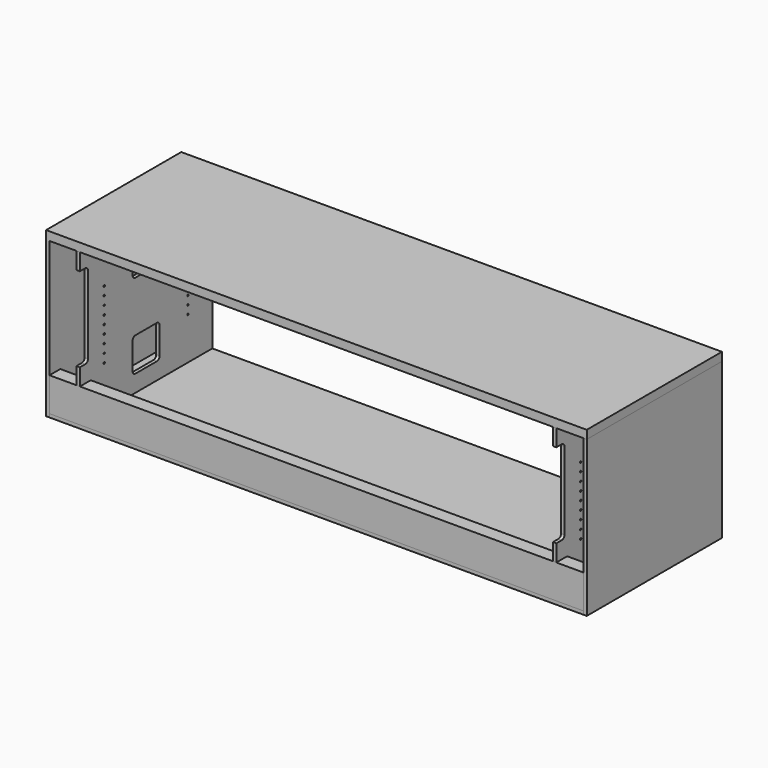
from build123d import *

# Parameters (mm, degrees)
F0_W      = 1600
F0_H      = 500
F1_DEPTH  = 25
F3_W      = 1580
F3_H      = 490
F4_DEPTH  = 10
F5_W      = 10
F5_H      = 500
F6_DEPTH  = 460
F7_W      = 10
F7_H      = 500
F8_DEPTH  = 460
F9_W      = 40
F9_H      = 100
F10_DEPTH = 1580
F11_W     = 10
F11_H     = 450
F12_DEPTH = 450
F13_W     = 10
F13_H     = 350
F14_DEPTH = 40
F16_W     = 30
F16_H     = 250
F17_DEPTH = 100.001
F18_R     = 10
F20_DEPTH = 100.001
F21_R     = 2.5
F22_DEPTH = 100.001


with BuildPart() as f1:
    # F0 (on Top) → F1 (new body)
    with BuildSketch(Plane.XY):
        with Locations((800, 250)):
            Rectangle(F0_W, F0_H)
    extrude(amount=F1_DEPTH)

    # F5 (on face) → F6 (join, through all)
    with BuildSketch(Plane.XY):
        with Locations((5, 250)):
            Rectangle(F5_W, F5_H)
    extrude(amount=-F6_DEPTH)


with BuildPart() as f4:
    # F3 (on offset) → F4 (new body)
    with BuildSketch(Plane.XY.offset(-460)):
        with Locations((800, 245)):
            Rectangle(F3_W, F3_H)
    extrude(amount=F4_DEPTH)


with BuildPart() as f8:
    # F7 (on face) → F8 (new body, through all)
    with BuildSketch(Plane.XY):
        with Locations((1595, 250)):
            Rectangle(F7_W, F7_H)
    extrude(amount=-F8_DEPTH)


with BuildPart() as f10:
    # F9 (on face) → F10 (new body, through all)
    with BuildSketch(Plane.YZ.offset(10)):
        with Locations((20, -400)):
            Rectangle(F9_W, F9_H)
    extrude(amount=F10_DEPTH)


with BuildPart() as f12:
    # F11 (on face) → F12 (new body, through all)
    with BuildSketch(Plane.XY.offset(-450)):
        with Locations((95, 265)):
            Rectangle(F11_W, F11_H)
    extrude(amount=F12_DEPTH)

    # F13 (on face) → F14 (join, through all)
    with BuildSketch(Plane.XZ.offset(-40)):
        with Locations((95, -175)):
            Rectangle(F13_W, F13_H)
    extrude(amount=F14_DEPTH)

    # F15: union 

    # F16 (on face) → F17 (cut, through all)
    with BuildSketch(Plane.YZ.offset(100)):
        with Locations((15, -175)):
            Rectangle(F16_W, F16_H)
    extrude(amount=-F17_DEPTH, mode=Mode.SUBTRACT)

    # F18
    f18_edges = [f12.edges().sort_by_distance(p)[0] for p in [
        (95, 30, -50),
        (95, 30, -300),
    ]]
    fillet(f18_edges, radius=F18_R)

    # F19 (on face) → F20 (cut, through all)
    with BuildSketch(Plane.YZ.offset(100)):
        with BuildLine():
            Line((285, -50), (205, -50))
            ThreePointArc((205, -50), (197.9289321881, -52.9289321881), (195, -60))
            Line((195, -60), (195, -140))
            ThreePointArc((195, -140), (197.9289321881, -147.0710678119), (205, -150))
            Line((205, -150), (285, -150))
            ThreePointArc((285, -150), (292.0710678119, -147.0710678119), (295, -140))
            Line((295, -140), (295, -60))
            ThreePointArc((295, -60), (292.0710678119, -52.9289321881), (285, -50))
        make_face()
        with BuildLine():
            Line((285, -300), (205, -300))
            ThreePointArc((205, -300), (197.9289321881, -302.9289321881), (195, -310))
            Line((195, -310), (195, -390))
            ThreePointArc((195, -390), (197.9289321881, -397.0710678119), (205, -400))
            Line((205, -400), (285, -400))
            ThreePointArc((285, -400), (292.0710678119, -397.0710678119), (295, -390))
            Line((295, -390), (295, -310))
            ThreePointArc((295, -310), (292.0710678119, -302.9289321881), (285, -300))
        make_face()
    extrude(amount=-F20_DEPTH, mode=Mode.SUBTRACT)

    # F21 (on face) → F22 (cut, through all)
    with BuildSketch(Plane.YZ.offset(100)):
        with Locations((90, -325)):
            Circle(F21_R)
        with Locations((90, -300)):
            Circle(F21_R)
        with Locations((90, -275)):
            Circle(F21_R)
        with Locations((90, -250)):
            Circle(F21_R)
        with Locations((90, -225)):
            Circle(F21_R)
        with Locations((90, -200)):
            Circle(F21_R)
        with Locations((90, -175)):
            Circle(F21_R)
        with Locations((90, -150)):
            Circle(F21_R)
        with Locations((90, -125)):
            Circle(F21_R)
        with Locations((400, -325)):
            Circle(F21_R)
        with Locations((400, -300)):
            Circle(F21_R)
        with Locations((400, -275)):
            Circle(F21_R)
        with Locations((400, -250)):
            Circle(F21_R)
        with Locations((400, -225)):
            Circle(F21_R)
        with Locations((400, -200)):
            Circle(F21_R)
        with Locations((400, -175)):
            Circle(F21_R)
        with Locations((400, -150)):
            Circle(F21_R)
        with Locations((400, -125)):
            Circle(F21_R)
    extrude(amount=-F22_DEPTH, mode=Mode.SUBTRACT)


with BuildPart() as f24_1:
    # F24: instance of F12
    add(f12.part.mirror(Plane(origin=(800, 250, -230), x_dir=(0, 1, 0), z_dir=(1, 0, 0))))


solid = Compound([f1.part, f4.part, f8.part, f10.part, f12.part, f24_1.part])
